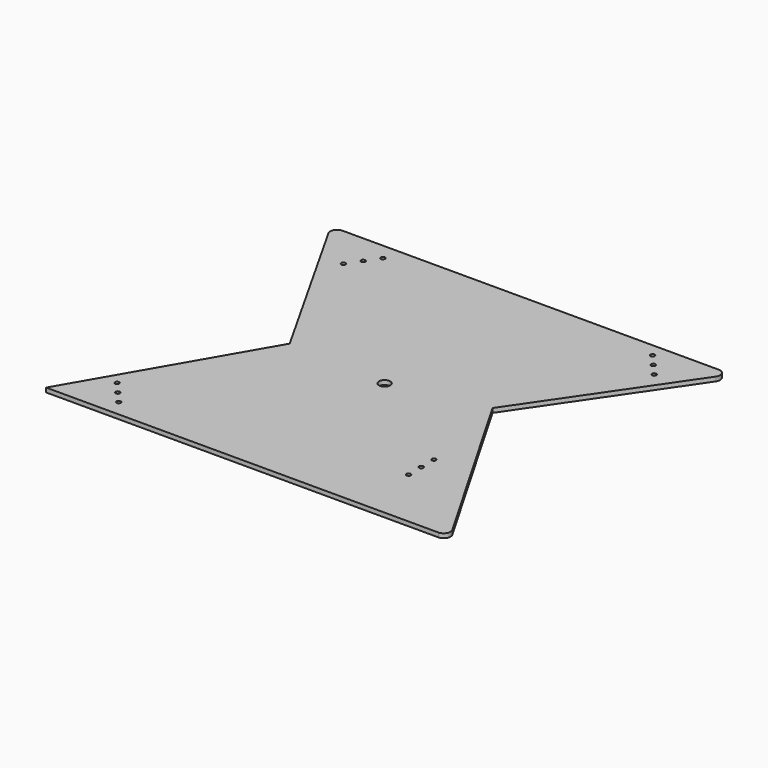
from build123d import *

# Parameters (mm, degrees)
F0_R     = 1.6
F0_R_2   = 4.15
F1_DEPTH = 3.2
F2_R     = 5


# Not quite as in the source:
# - a feature names something its author has since deleted; it is built from what else it names


with BuildPart() as f1:
    # F0 (on Top) → F1 (new body)
    with BuildSketch(Plane.XY):
        Polygon((-147.5119216098, 134.4644985315), (-74.1683009258, 4.5805452964), (-5.9605e-06, 133.0438004871), (68.2159057757, 14.8903754755), (149.9999940395, 134.4644985315), align=None)
        with BuildLine():
            Line((-96.8504283589, 106.236077336), (-103.5946726395, 96.3105965374))
            Line((-103.5946726395, 96.3105965374), (-111.1628517485, 101.4530828014))
            ThreePointArc((-111.1628517485, 101.4530828014), (-113.385481759, 101.0289179323), (-113.8096466281, 103.2515479429))
            Line((-113.8096466281, 103.2515479429), (-121.377825737, 108.3940342069))
            Line((-121.377825737, 108.3940342069), (-114.6335814564, 118.3195150055))
            Line((-114.6335814564, 118.3195150055), (-107.8893371757, 128.244995804))
            Line((-107.8893371757, 128.244995804), (-100.3211580668, 123.10250954))
            ThreePointArc((-100.3211580668, 123.10250954), (-98.5273543684, 123.7325637154), (-97.397760627, 122.2032769693))
            ThreePointArc((-97.397760627, 122.2032769693), (-97.4684738809, 121.7328707107), (-97.6743631872, 121.3040443985))
            Line((-97.6743631872, 121.3040443985), (-90.1061840783, 116.1615581346))
            Line((-90.1061840783, 116.1615581346), (-96.8504283589, 106.236077336))
        make_face(mode=Mode.SUBTRACT)
        with BuildLine():
            Line((115.3912264438, 122.4205616549), (123.2329658209, 113.3372184629))
            Line((123.2329658209, 113.3372184629), (116.306916637, 107.3578921879))
            ThreePointArc((116.306916637, 107.3578921879), (116.5954341459, 106.870099346), (116.6958042114, 106.3123269377))
            ThreePointArc((116.6958042114, 106.3123269377), (115.6535766198, 104.8126970032), (113.8846917858, 105.2667616874))
            Line((113.8846917858, 105.2667616874), (106.958642602, 99.2874354124))
            Line((106.958642602, 99.2874354124), (99.1169032249, 108.3707786044))
            Line((99.1169032249, 108.3707786044), (91.2751638479, 117.4541217963))
            Line((91.2751638479, 117.4541217963), (98.2012130318, 123.4334480713))
            ThreePointArc((98.2012130318, 123.4334480713), (98.3667602071, 125.6901257472), (100.6234378829, 125.5245785718))
            Line((100.6234378829, 125.5245785718), (107.5494870668, 131.5039048468))
            Line((107.5494870668, 131.5039048468), (115.3912264438, 122.4205616549))
        make_face(mode=Mode.SUBTRACT)
        Polygon((-74.1683009258, 4.5805452964), (-5.9605e-06, -126.7638206482), (49.5534456811, -23.8632776696), (68.2159057757, 14.8903754755), (-5.9605e-06, 133.0438004871), align=None)
        with BuildLine():
            ThreePointArc((55, 0), (53.6210756721, -12.2384739151), (49.5534456811, -23.8632776696))
            ThreePointArc((49.5534456811, -23.8632776696), (-53.6210756721, 12.2384739151), (55, 0))
        make_face(mode=Mode.SUBTRACT)
        Polygon((49.5534456811, -23.8632776696), (-5.9605e-06, -126.7638206482), (149.9999940395, -126.7638206482), (68.2159057757, 14.8903754755), align=None)
        with Locations((82.4472344942, -80.8260182953)):
            Circle(F0_R, mode=Mode.SUBTRACT)
        with Locations((82.2787740784, -68.8272008082)):
            Circle(F0_R, mode=Mode.SUBTRACT)
        with Locations((82.1103136625, -56.8283833211)):
            Circle(F0_R, mode=Mode.SUBTRACT)
        Polygon((-74.1683009258, 4.5805452964), (-150.0000059605, -126.7638206482), (-5.9605e-06, -126.7638206482), align=None)
        with BuildLine():
            Line((-105.4957706959, -98.6149983111), (-97.6540313188, -107.698341503))
            Line((-97.6540313188, -107.698341503), (-104.5800805027, -113.677667778))
            ThreePointArc((-104.5800805027, -113.677667778), (-104.2915629938, -114.1654606199), (-104.1911929283, -114.7232330283))
            ThreePointArc((-104.1911929283, -114.7232330283), (-105.2334205199, -116.2228629628), (-107.0023053539, -115.7687982785))
            Line((-107.0023053539, -115.7687982785), (-113.9283545378, -121.7481245535))
            Line((-113.9283545378, -121.7481245535), (-121.7700939148, -112.6647813616))
            Line((-121.7700939148, -112.6647813616), (-129.6118332918, -103.5814381696))
            Line((-129.6118332918, -103.5814381696), (-122.685784108, -97.6021118946))
            ThreePointArc((-122.685784108, -97.6021118946), (-122.5202369326, -95.3454342188), (-120.2635592568, -95.5109813941))
            Line((-120.2635592568, -95.5109813941), (-113.3375100729, -89.5316551191))
            Line((-113.3375100729, -89.5316551191), (-105.4957706959, -98.6149983111))
        make_face(mode=Mode.SUBTRACT)
        with BuildLine():
            ThreePointArc((55, 0), (-53.6210756721, 12.2384739151), (49.5534456811, -23.8632776696))
            ThreePointArc((49.5534456811, -23.8632776696), (53.6210756721, -12.2384739151), (55, 0))
        make_face()
        Circle(F0_R_2, mode=Mode.SUBTRACT)
        with BuildLine():
            Line((-111.1628517485, 101.4530828014), (-103.5946726395, 96.3105965374))
            Line((-103.5946726395, 96.3105965374), (-96.8504283589, 106.236077336))
            Line((-96.8504283589, 106.236077336), (-104.4186074678, 111.3785636))
            ThreePointArc((-104.4186074678, 111.3785636), (-105.4420750524, 110.7061594182), (-106.6412374784, 110.9543987309))
            Line((-106.6412374784, 110.9543987309), (-111.5870166175, 103.6757128119))
            ThreePointArc((-111.5870166175, 103.6757128119), (-111.0722527043, 103.1010569453), (-110.8862491883, 102.3523153721))
            ThreePointArc((-110.8862491883, 102.3523153721), (-110.9569624422, 101.8819091135), (-111.1628517485, 101.4530828014))
        make_face()
        with BuildLine():
            Line((-104.4186074678, 111.3785636), (-96.8504283589, 106.236077336))
            Line((-96.8504283589, 106.236077336), (-90.1061840783, 116.1615581346))
            Line((-90.1061840783, 116.1615581346), (-97.6743631872, 121.3040443985))
            ThreePointArc((-97.6743631872, 121.3040443985), (-98.6978307717, 120.6316402168), (-99.8969931977, 120.8798795295))
            Line((-99.8969931977, 120.8798795295), (-104.8427723369, 113.6011936105))
            ThreePointArc((-104.8427723369, 113.6011936105), (-104.3280084237, 113.0265377439), (-104.1420049076, 112.2777961707))
            ThreePointArc((-104.1420049076, 112.2777961707), (-104.2127181615, 111.8073899121), (-104.4186074678, 111.3785636))
        make_face()
        with BuildLine():
            Line((-121.377825737, 108.3940342069), (-113.8096466281, 103.2515479429))
            ThreePointArc((-113.8096466281, 103.2515479429), (-112.7861790435, 103.9239521247), (-111.5870166175, 103.6757128119))
            Line((-111.5870166175, 103.6757128119), (-106.6412374784, 110.9543987309))
            ThreePointArc((-106.6412374784, 110.9543987309), (-107.3136416602, 111.9778663155), (-107.0654023474, 113.1770287415))
            Line((-107.0654023474, 113.1770287415), (-114.6335814564, 118.3195150055))
            Line((-114.6335814564, 118.3195150055), (-121.377825737, 108.3940342069))
        make_face()
        with BuildLine():
            Line((-107.8893371757, 128.244995804), (-114.6335814564, 118.3195150055))
            Line((-114.6335814564, 118.3195150055), (-107.0654023474, 113.1770287415))
            ThreePointArc((-107.0654023474, 113.1770287415), (-106.0419347629, 113.8494329232), (-104.8427723369, 113.6011936105))
            Line((-104.8427723369, 113.6011936105), (-99.8969931977, 120.8798795295))
            ThreePointArc((-99.8969931977, 120.8798795295), (-100.5693973795, 121.903347114), (-100.3211580668, 123.10250954))
            Line((-100.3211580668, 123.10250954), (-107.8893371757, 128.244995804))
        make_face()
        with BuildLine():
            Line((-104.5800805027, -113.677667778), (-97.6540313188, -107.698341503))
            Line((-97.6540313188, -107.698341503), (-105.4957706959, -98.6149983111))
            Line((-105.4957706959, -98.6149983111), (-112.4218198797, -104.594324586))
            ThreePointArc((-112.4218198797, -104.594324586), (-112.1333023708, -105.082117428), (-112.0329323053, -105.6398898363))
            ThreePointArc((-112.0329323053, -105.6398898363), (-112.1781291571, -106.30588368), (-112.5873670551, -106.8510022619))
            Line((-112.5873670551, -106.8510022619), (-106.8367581786, -113.5121206027))
            ThreePointArc((-106.8367581786, -113.5121206027), (-105.674133398, -113.1275209407), (-104.5800805027, -113.677667778))
        make_face()
        with BuildLine():
            Line((-112.4218198797, -104.594324586), (-105.4957706959, -98.6149983111))
            Line((-105.4957706959, -98.6149983111), (-113.3375100729, -89.5316551191))
            Line((-113.3375100729, -89.5316551191), (-120.2635592568, -95.5109813941))
            ThreePointArc((-120.2635592568, -95.5109813941), (-119.9750417479, -95.998774236), (-119.8746716824, -96.5565466444))
            ThreePointArc((-119.8746716824, -96.5565466444), (-120.0198685341, -97.222540488), (-120.4291064321, -97.76765907))
            Line((-120.4291064321, -97.76765907), (-114.6784975556, -104.4287774107))
            ThreePointArc((-114.6784975556, -104.4287774107), (-113.5158727751, -104.0441777488), (-112.4218198797, -104.594324586))
        make_face()
        with BuildLine():
            ThreePointArc((-107.0023053539, -115.7687982785), (-107.3869050159, -114.606173498), (-106.8367581786, -113.5121206027))
            Line((-106.8367581786, -113.5121206027), (-112.5873670551, -106.8510022619))
            ThreePointArc((-112.5873670551, -106.8510022619), (-113.7499918356, -107.2356019239), (-114.8440447309, -106.6854550866))
            Line((-114.8440447309, -106.6854550866), (-121.7700939148, -112.6647813616))
            Line((-121.7700939148, -112.6647813616), (-113.9283545378, -121.7481245535))
            Line((-113.9283545378, -121.7481245535), (-107.0023053539, -115.7687982785))
        make_face()
        with BuildLine():
            ThreePointArc((-114.8440447309, -106.6854550866), (-115.2286443929, -105.522830306), (-114.6784975556, -104.4287774107))
            Line((-114.6784975556, -104.4287774107), (-120.4291064321, -97.76765907))
            ThreePointArc((-120.4291064321, -97.76765907), (-121.5917312126, -98.1522587319), (-122.685784108, -97.6021118946))
            Line((-122.685784108, -97.6021118946), (-129.6118332918, -103.5814381696))
            Line((-129.6118332918, -103.5814381696), (-121.7700939148, -112.6647813616))
            Line((-121.7700939148, -112.6647813616), (-114.8440447309, -106.6854550866))
        make_face()
        with BuildLine():
            Line((116.306916637, 107.3578921879), (123.2329658209, 113.3372184629))
            Line((123.2329658209, 113.3372184629), (115.3912264438, 122.4205616549))
            Line((115.3912264438, 122.4205616549), (108.46517726, 116.4412353799))
            ThreePointArc((108.46517726, 116.4412353799), (108.7536947689, 115.953442538), (108.8540648344, 115.3956701296))
            ThreePointArc((108.8540648344, 115.3956701296), (108.7088679827, 114.729676286), (108.2996300847, 114.184557704))
            Line((108.2996300847, 114.184557704), (114.0502389611, 107.5234393633))
            ThreePointArc((114.0502389611, 107.5234393633), (115.2128637417, 107.9080390252), (116.306916637, 107.3578921879))
        make_face()
        with BuildLine():
            Line((108.46517726, 116.4412353799), (115.3912264438, 122.4205616549))
            Line((115.3912264438, 122.4205616549), (107.5494870668, 131.5039048468))
            Line((107.5494870668, 131.5039048468), (100.6234378829, 125.5245785718))
            ThreePointArc((100.6234378829, 125.5245785718), (100.9119553919, 125.0367857299), (101.0123254573, 124.4790133216))
            ThreePointArc((101.0123254573, 124.4790133216), (100.8671286056, 123.8130194779), (100.4578907076, 123.267900896))
            Line((100.4578907076, 123.267900896), (106.2084995841, 116.6067825552))
            ThreePointArc((106.2084995841, 116.6067825552), (107.3711243647, 116.9913822172), (108.46517726, 116.4412353799))
        make_face()
        with BuildLine():
            ThreePointArc((113.8846917858, 105.2667616874), (113.5000921239, 106.4293864679), (114.0502389611, 107.5234393633))
            Line((114.0502389611, 107.5234393633), (108.2996300847, 114.184557704))
            ThreePointArc((108.2996300847, 114.184557704), (107.1370053041, 113.7999580421), (106.0429524088, 114.3501048793))
            Line((106.0429524088, 114.3501048793), (99.1169032249, 108.3707786044))
            Line((99.1169032249, 108.3707786044), (106.958642602, 99.2874354124))
            Line((106.958642602, 99.2874354124), (113.8846917858, 105.2667616874))
        make_face()
        with BuildLine():
            ThreePointArc((106.0429524088, 114.3501048793), (105.6583527468, 115.5127296599), (106.2084995841, 116.6067825552))
            Line((106.2084995841, 116.6067825552), (100.4578907076, 123.267900896))
            ThreePointArc((100.4578907076, 123.267900896), (99.2952659271, 122.883301234), (98.2012130318, 123.4334480713))
            Line((98.2012130318, 123.4334480713), (91.2751638479, 117.4541217963))
            Line((91.2751638479, 117.4541217963), (99.1169032249, 108.3707786044))
            Line((99.1169032249, 108.3707786044), (106.0429524088, 114.3501048793))
        make_face()
    extrude(amount=F1_DEPTH)

    # F2
    f2_edges = [f1.edges().sort_by_distance(p)[0] for p in [
        (149.999994, -126.763821, 1.6),
        (149.999994, 134.464499, 1.6),
        (-147.511922, 134.464499, 1.6),
    ]]
    fillet(f2_edges, radius=F2_R)


solid = f1.part
